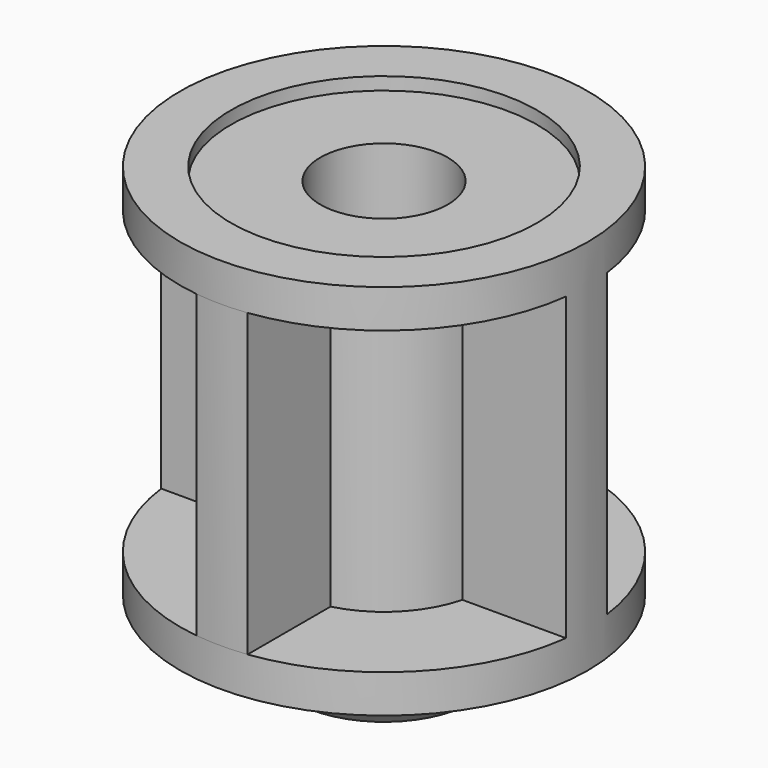
from build123d import *

# Parameters (mm, degrees)
F0_R             = 12.7
F0_R_2           = 3.96875
F1_DEPTH         = 1.5875
F2_R             = 12.7
F2_R_2           = 9.525
F3_DEPTH         = 0.79375
F4_R             = 6.35
F4_R_2           = 3.96875
F5_DEPTH         = 18.7244736
F6_R             = 12.7
F6_R_2           = 3.96875
F7_DEPTH         = 1.5875
F8_R             = 12.7
F8_R_2           = 9.525
F9_DEPTH         = 0.79375
F11_DEPTH        = 18.7244736
F11_COPIES_COUNT = 4
F12_R            = 7.14375
F12_R_2          = 3.96875
F13_DEPTH        = 4.85775
F14_SIZE         = 1.5875


# Not quite as in the source:
# - a length typed as a fraction of an inch, garbled in the dataset ("3 / 203.2 mm" for 3/8 in), is restored
# - a pattern or mirror of a feature is missing from the dataset's text; its kind, count and spacing are read off the source's solid


with BuildPart() as f1:
    # F0 (on Top) → F1 (new body)
    with BuildSketch(Plane.XY):
        Circle(F0_R)
        Circle(F0_R_2, mode=Mode.SUBTRACT)
    extrude(amount=F1_DEPTH)

    # F2 (on face) → F3 (join)
    with BuildSketch(Plane(origin=(0, 0, 0), x_dir=(1, 0, 0), z_dir=(0, 0, -1))):
        Circle(F2_R)
        Circle(F2_R_2, mode=Mode.SUBTRACT)
    extrude(amount=F3_DEPTH)

    # F4 (on face) → F5 (join)
    with BuildSketch(Plane.XY.offset(1.5875)):
        Circle(F4_R)
        Circle(F4_R_2, mode=Mode.SUBTRACT)
    extrude(amount=F5_DEPTH)

    # F6 (on face) → F7 (join)
    with BuildSketch(Plane.XY.offset(20.3119736)):
        Circle(F6_R)
        Circle(F6_R_2, mode=Mode.SUBTRACT)
    extrude(amount=F7_DEPTH)

    # F8 (on face) → F9 (join)
    with BuildSketch(Plane.XY.offset(21.8994736)):
        Circle(F8_R)
        Circle(F8_R_2, mode=Mode.SUBTRACT)
    extrude(amount=F9_DEPTH)

    # F10 (on face) → F11 (join, through all)
    with BuildSketch(Plane.XY.offset(1.5875)):
        with BuildLine():
            Line((1.5875, -12.6003906189), (1.5875, -6.1483610621))
            ThreePointArc((1.5875, -6.1483610621), (0, -6.35), (-1.5875, -6.1483610621))
            Line((-1.5875, -6.1483610621), (-1.5875, -12.6003906189))
            ThreePointArc((-1.5875, -12.6003906189), (0, -12.7), (1.5875, -12.6003906189))
        make_face()
    f11 = extrude(amount=F11_DEPTH)

    # F11_copies: F11 ×4 about axis
    f11_copies_axis = Axis((0, 0, 0), (0, 0, 1))
    for i in range(1, F11_COPIES_COUNT):
        add(f11.rotate(f11_copies_axis, i * 360 / F11_COPIES_COUNT))

    # F12 (on face) → F13 (join)
    with BuildSketch(Plane(origin=(0, 0, 0), x_dir=(1, 0, 0), z_dir=(0, 0, -1))):
        Circle(F12_R)
        Circle(F12_R_2, mode=Mode.SUBTRACT)
    extrude(amount=F13_DEPTH)

    # F14
    f14_edges = [f1.edges().sort_by_distance(p)[0] for p in [
        (-7.14375, 0, -4.85775),
    ]]
    chamfer(f14_edges, length=F14_SIZE)


solid = f1.part
